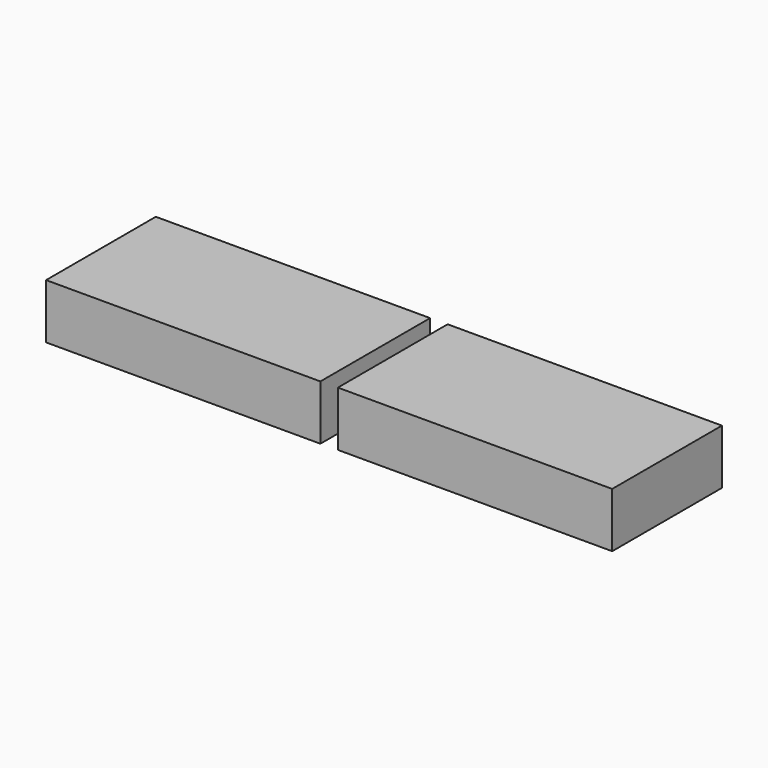
from build123d import *

# Parameters (mm, degrees)
F1_W     = 1270
F1_H     = 635
F2_DEPTH = 254


# Not quite as in the source:
# - a variable given as a bare number and used for a length is read in inches; the dataset says mm whatever the document's units were


with BuildPart() as f2:
    # F1 (on Top) → F2 (new body)
    with BuildSketch(Plane.XY):
        with Locations((-635, 317.5)):
            Rectangle(F1_W, F1_H)
    extrude(amount=F2_DEPTH)


with BuildPart() as f2b:
    # F1 (on Top) → F2, piece 2 (new body)
    with BuildSketch(Plane.XY):
        with Locations((714.5902907848, 319.2255449295)):
            Rectangle(F1_W, F1_H)
    extrude(amount=F2_DEPTH)


solid = Compound([f2.part, f2b.part])
